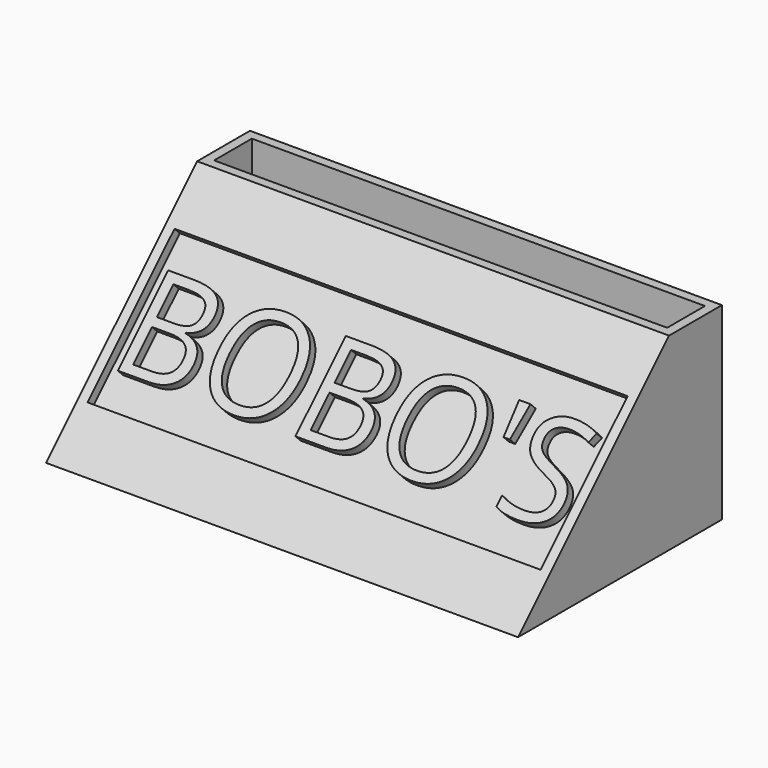
from build123d import *

# Parameters (mm, degrees)
F0_W         = 100
F0_H         = 54
F1_DEPTH     = 40
F3_DEPTH     = 100
F4_W         = 96
F4_H         = 32.5685424949
F5_DEPTH     = 2
F6_W         = 96
F6_H         = 10
F7_DEPTH     = 18
F8_TEXT_SIZE = 26.370230482
F9_DEPTH     = 2


# Not quite as in the source:
# - a feature names something its author has since deleted; it is built from what else it names
# - Text() gives the source's letters only with a copy of the font that has no kerning and outlines rounded to 1/6400 em; it was checked with that copy


with BuildPart() as f1:
    # F0 (on Top) → F1 (new body)
    with BuildSketch(Plane.XY):
        Rectangle(F0_W, F0_H)
    extrude(amount=F1_DEPTH)

    # F2 (on face) → F3 (cut, through all)
    with BuildSketch(Plane(origin=(-50, 0, 0), x_dir=(0, -1, 0), z_dir=(-1, 0, 0))):
        Polygon((27, 40), (-13, 40), (27, 0), align=None)
    extrude(amount=-F3_DEPTH, mode=Mode.SUBTRACT)

    # F4 (on face) → F5 (cut)
    with BuildSketch(Plane(origin=(0, -13.5, 13.5), x_dir=(1, 0, 0), z_dir=(0, -0.7071067812, 0.7071067812))):
        with Locations((0, 9.1923881554)):
            Rectangle(F4_W, F4_H)
    extrude(amount=-F5_DEPTH, mode=Mode.SUBTRACT)

    # F6 (on face) → F7 (cut)
    with BuildSketch(Plane.XY.offset(40)):
        with Locations((0, 20)):
            Rectangle(F6_W, F6_H)
    extrude(amount=-F7_DEPTH, mode=Mode.SUBTRACT)

    # F8 (on face) → F9 (join)
    with BuildSketch(Plane(origin=(0, -12.0857864376, 12.0857864376), x_dir=(1, 0, 0), z_dir=(0, -0.7071067812, 0.7071067812))):
        with Locations((-48, -0.3008948181)):
            Text("BOBO'S", F8_TEXT_SIZE, font='Open Sans', text_align=(TextAlign.LEFT, TextAlign.BOTTOM))
    extrude(amount=F9_DEPTH)


solid = f1.part
